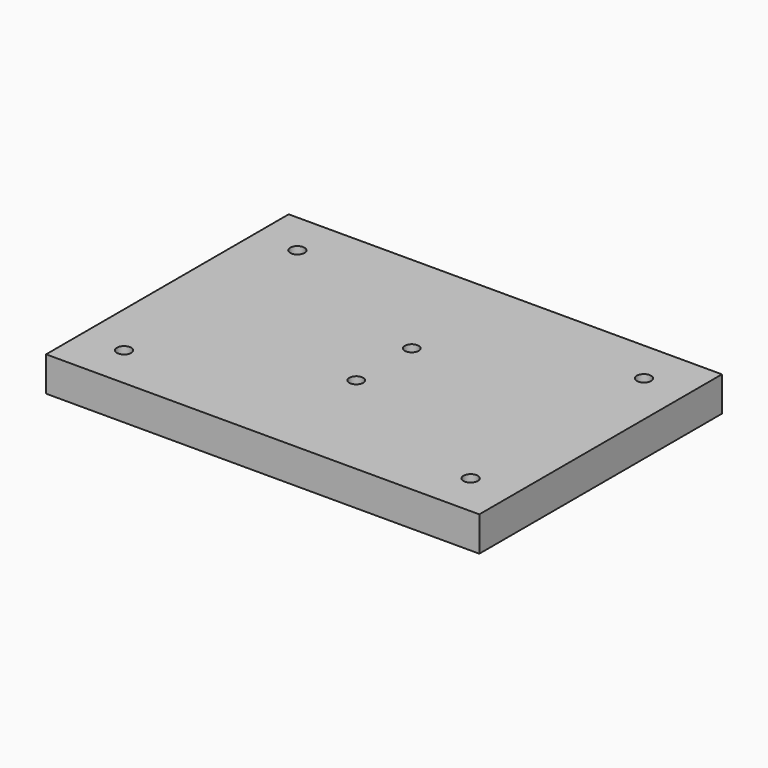
from build123d import *

# Parameters (mm, degrees)
F0_W     = 100
F0_H     = 70
F1_DEPTH = 4
F3_D     = 3.3
F4_D     = 3.2


with BuildPart() as f1:
    # F0 (on Top) → F1 (new body, symmetric)
    with BuildSketch(Plane.XY):
        Rectangle(F0_W, F0_H)
    extrude(amount=F1_DEPTH, both=True)

    # F3 (through all)
    with Locations(Plane.XY.offset(4)):
        with Locations((40, 25), (40, -25), (-40, -25), (-40, 25)):
            Hole(F3_D / 2)

    # F4 (through all)
    with Locations(Plane.XY.offset(4)):
        with Locations((0, 8), (0, -8)):
            Hole(F4_D / 2)


solid = f1.part
